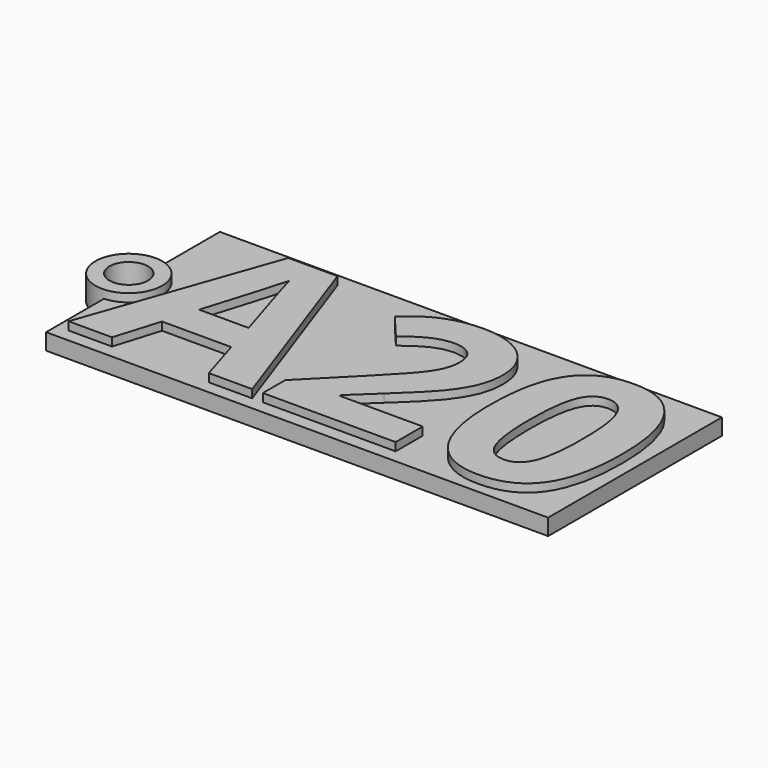
from build123d import *

# Parameters (mm, degrees)
F0_TEXT_SIZE = 82.9065529009
F1_DEPTH     = 7.62
F2_W         = 156.4105376601
F2_H         = 67.6776319742
F3_DEPTH     = 5.08
F4_R         = 10.39685297
F5_DEPTH     = 7.62
F6_R         = 6.0191130335
F7_DEPTH     = 25.4


# Not quite as in the source:
# - Text() gives the source's letters only with a copy of the font that has no kerning and outlines rounded to 1/6400 em; it was checked with that copy


with BuildPart() as f1:
    # F0 (on Top) → F1 (new body)
    with BuildSketch(Plane.XY):
        with Locations((-77.2482231259, -18.3118903078)):
            Text('A20', F0_TEXT_SIZE, font='Open Sans', font_style=FontStyle.BOLD, text_align=(TextAlign.LEFT, TextAlign.BOTTOM))
    extrude(amount=F1_DEPTH)


with BuildPart() as f3:
    # F2 (on Top) → F3 (new body)
    with BuildSketch(Plane.XY):
        with Locations((-2.7800314128, 11.4299990237)):
            Rectangle(F2_W, F2_H)
    extrude(amount=F3_DEPTH)

    # F4 (on Top) → F5 (join)
    with BuildSketch(Plane.XY):
        with Locations((-81.5566256642, 10.5149094015)):
            Circle(F4_R)
    extrude(amount=F5_DEPTH)

    # F6 (on face) → F7 (cut)
    with BuildSketch(Plane.XY.offset(7.62)):
        with Locations((-81.5566256642, 10.5149094015)):
            Circle(F6_R)
    extrude(amount=-F7_DEPTH, mode=Mode.SUBTRACT)


solid = Compound([f1.part, f3.part])
